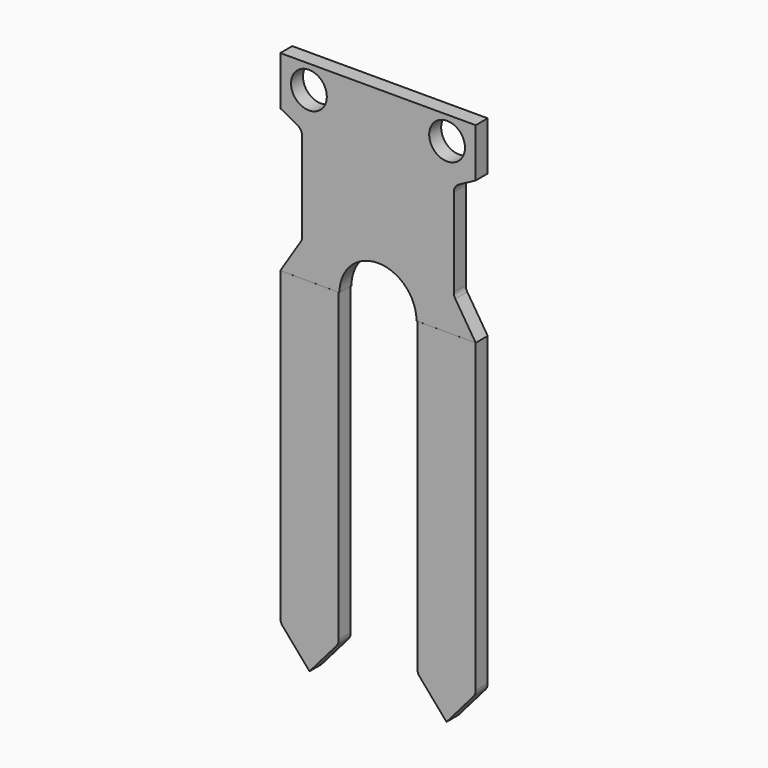
from build123d import *

# Parameters (mm, degrees)
F1_DEPTH = 1.55
F0_R     = 1.85
F2_R     = 1
F2_2_R   = 1
F2_3_R   = 1


# Not quite as in the source:
# - ends of sketch curves that miss each other by under 0.0002 mm in the source are joined


with BuildPart() as f1:
    # F0 (on Front) → F1 (new body)
    with BuildSketch(Plane.XZ):
        Polygon((-4.0597100742, -9.902607639), (-10.1, -9.9000012899), (-10.1, -41.8800012899), (-7.0798584417, -45.3703802887), (-4.0597100742, -41.8800014933), align=None)
    extrude(amount=F1_DEPTH)

    # F2#2
    f2_2_edges = [f1.edges().sort_by_distance(p)[0] for p in [
        (-10.1, -0.775, -41.880001),
        (-4.05971, -0.775, -41.880001),
    ]]
    fillet(f2_2_edges, radius=F2_2_R)


with BuildPart() as f1b:
    # F0 (on Front) → F1, piece 2 (new body)
    with BuildSketch(Plane.XZ):
        Polygon((10.1, -41.8800012899), (10.1, -9.9000012899), (4.0597100742, -9.902607639), (4.0597100742, -41.8800014933), (7.0798584417, -45.3703802887), align=None)
        Polygon((4.0597100742, -9.902607639), (10.1, -9.9000012899), (4.0597100742, -9.9000005185), align=None)
    extrude(amount=F1_DEPTH)

    # F2#3
    f2_3_edges = [f1b.edges().sort_by_distance(p)[0] for p in [
        (4.05971, -0.775, -41.880001),
        (10.1, -0.775, -41.880001),
    ]]
    fillet(f2_3_edges, radius=F2_3_R)


with BuildPart() as f1c:
    # F0 (on Front) → F1, piece 3 (new body)
    with BuildSketch(Plane.XZ):
        with BuildLine():
            Line((10.1, 9.9000012899), (-10.1, 9.899998069))
            Line((-10.1, 9.899998069), (-10.099999198, 4.869998069))
            Line((-10.099999198, 4.869998069), (-7.8321473486, 3.6609703649))
            Line((-7.8321473486, 3.6609703649), (-7.8321473486, -6.3390296351))
            Line((-7.8321473486, -6.3390296351), (-10.1, -9.9000012899))
            Line((-10.1, -9.9000012899), (-4.0597100742, -9.9000005185))
            Line((-4.0597100742, -9.9000005185), (-4.0597100742, -9.902607639))
            Line((-4.0597100742, -9.902607639), (-3.9800005697, -9.9026420332))
            ThreePointArc((-3.9800005697, -9.9026420332), (-0.0026423538, -5.9199991097), (3.9800005697, -9.8973573257))
            Line((3.9800005697, -9.8973573257), (10.1, -9.899998069))
            Line((10.1, -9.899998069), (7.8321473486, -6.3390296351))
            Line((7.8321473486, -6.3390296351), (7.8321473486, 3.6609703649))
            Line((7.8321473486, 3.6609703649), (10.099999198, 4.869998069))
            Line((10.099999198, 4.869998069), (10.1, 9.9000012899))
        make_face()
        with Locations((-7.1400015305, 7.489998541)):
            Circle(F0_R, mode=Mode.SUBTRACT)
        with Locations((7.1400015305, 7.489998541)):
            Circle(F0_R, mode=Mode.SUBTRACT)
    extrude(amount=F1_DEPTH)

    # F2
    f2_edges = [f1c.edges().sort_by_distance(p)[0] for p in [
        (7.832147, -0.775, 3.66097),
        (7.832147, -0.775, -6.33903),
        (-7.832147, -0.775, 3.66097),
        (-7.832147, -0.775, -6.33903),
    ]]
    fillet(f2_edges, radius=F2_R)


solid = Compound([f1.part, f1b.part, f1c.part])
